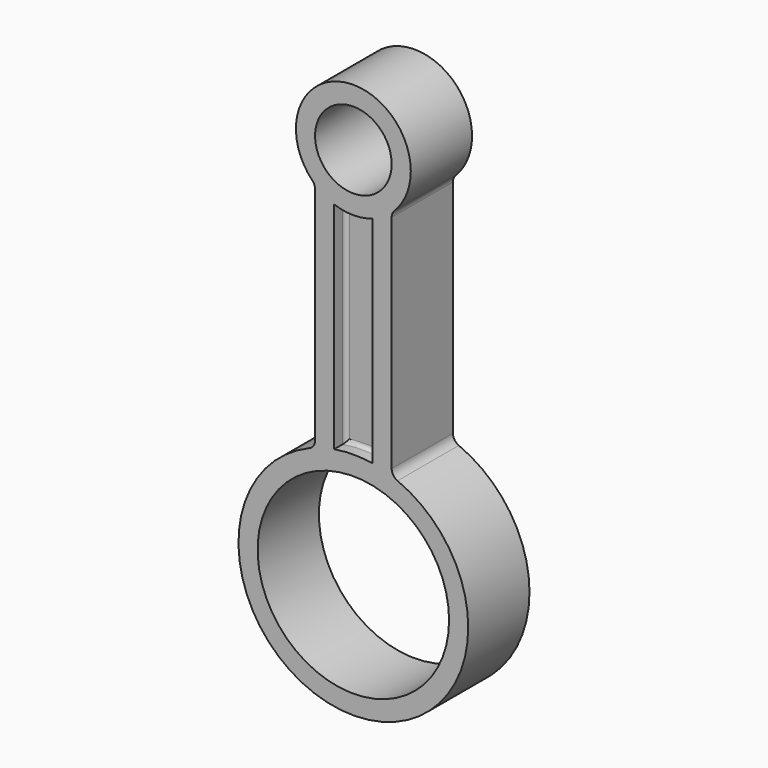
from build123d import *

# Parameters (mm, degrees)
F0_R     = 5.08
F0_R_2   = 12.7
F1_DEPTH = 5.08
F2_R     = 1.27
F4_DEPTH = 1.905
F5_R     = 0.508


# Not quite as in the source:
# - a pattern or mirror of a feature is missing from the dataset's text; its kind, count and spacing are read off the source's solid


with BuildPart() as f1:
    # F0 (on Front) → F1 (new body, symmetric)
    with BuildSketch(Plane.XZ):
        with BuildLine():
            ThreePointArc((5.08, 19.7203873372), (6.9560764803, 22.2891480267), (7.62, 25.4))
            ThreePointArc((7.62, 25.4), (-3.1108519733, 32.3560764803), (-5.08, 19.7203873372))
            ThreePointArc((-5.08, 19.7203873372), (0, 17.78), (5.08, 19.7203873372))
        make_face()
        with Locations((0, 25.4)):
            Circle(F0_R, mode=Mode.SUBTRACT)
        with BuildLine():
            ThreePointArc((5.08, 19.7203873372), (0, 17.78), (-5.08, 19.7203873372))
            Line((-5.08, 19.7203873372), (-5.08, -11.0315902063))
            ThreePointArc((-5.08, -11.0315902063), (0, -10.16), (5.08, -11.0315902063))
            Line((5.08, -11.0315902063), (5.08, 19.7203873372))
        make_face()
        with BuildLine():
            ThreePointArc((5.08, -11.0315902063), (0, -10.16), (-5.08, -11.0315902063))
            ThreePointArc((-5.08, -11.0315902063), (-8.7988181024, -37.8434078933), (15.24, -25.4))
            ThreePointArc((15.24, -25.4), (12.4434078933, -16.6011818976), (5.08, -11.0315902063))
        make_face()
        with Locations((0, -25.4)):
            Circle(F0_R_2, mode=Mode.SUBTRACT)
    extrude(amount=F1_DEPTH, both=True)

    # F2
    f2_edges = [f1.edges().sort_by_distance(p)[0] for p in [
        (-5.08, 0, 19.720387),
        (-5.08, 0, -11.03159),
        (5.08, 0, 19.720387),
        (5.08, 0, -11.03159),
    ]]
    fillet(f2_edges, radius=F2_R)

    # F3 (on face) → F4 (cut)
    with BuildSketch(Plane.XZ.offset(5.08)):
        with BuildLine():
            ThreePointArc((2.54, 18.2157951031), (0, 17.78), (-2.54, 18.2157951031))
            Line((-2.54, 18.2157951031), (-2.54, -10.3731573509))
            ThreePointArc((-2.54, -10.3731573509), (0, -10.16), (2.54, -10.3731573509))
            Line((2.54, -10.3731573509), (2.54, 18.2157951031))
        make_face()
    f4 = extrude(amount=-F4_DEPTH, mode=Mode.SUBTRACT)

    # F4_copies: F4 across plane
    add(f4.mirror(Plane.ZX), mode=Mode.SUBTRACT)

    # F5
    f5_edges = [f1.edges().sort_by_distance(p)[0] for p in [
        (-2.54, -3.175, 3.921319),
        (0, -3.175, 17.78),
        (2.54, -3.175, 3.921319),
        (0, -3.175, -10.16),
        (2.54, 4.1275, -10.373157),
        (2.54, 4.1275, 18.215795),
        (2.54, 3.175, 3.921319),
        (-2.54, 4.1275, 18.215795),
        (0, 3.175, 17.78),
        (-2.54, 4.1275, -10.373157),
        (-2.54, 3.175, 3.921319),
        (0, 3.175, -10.16),
    ]]
    fillet(f5_edges, radius=F5_R)


solid = f1.part
